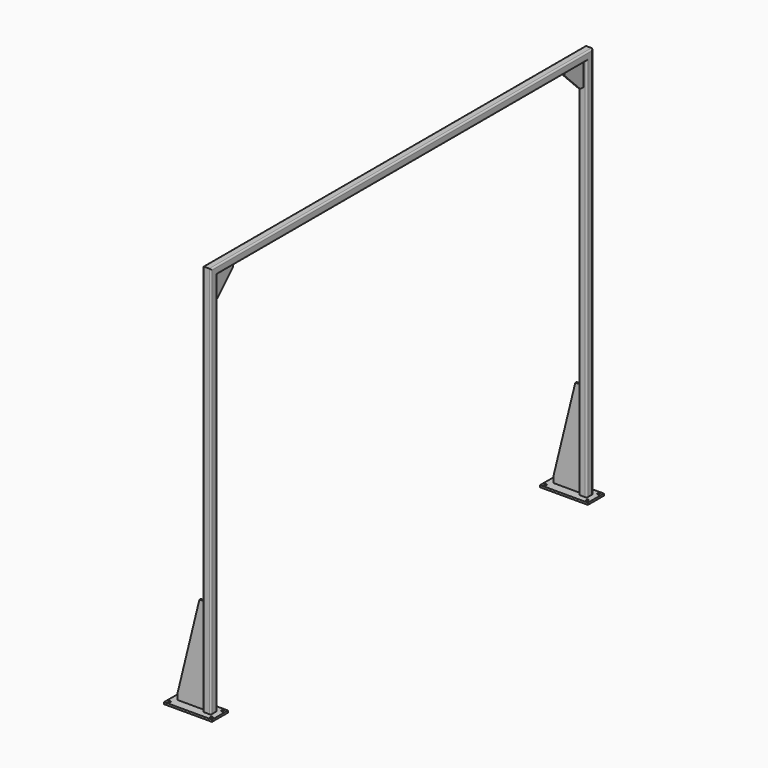
from build123d import *

# Parameters (mm, degrees)
F3_W      = 127
F3_H      = 127
F3_W_2    = 177.8
F4_DEPTH  = 12.7
F6_W      = 38.1
F6_H      = 38.1
F6_W_2    = 139.7
F6_H_2    = 571.5
F7_DEPTH  = 4.826
F9_D      = 14.2875
F13_DEPTH = 4.7625


# Not quite as in the source:
# - a length typed as a fraction of an inch, garbled in the dataset ("3 / 203.2 mm" for 3/8 in), is restored


with BuildPart() as f2:
    # F2: sweep along a path in F0
    with BuildLine(Plane.YZ) as f2_path:
        Line((-1524, 0), (-1524, 2501.9))
        Line((-1524, 2501.9), (1524, 2501.9))
        Line((1524, 2501.9), (1524, 0))
    # F1 (on Top) → F2 (sweep)
    with BuildSketch(Plane.XY):
        with BuildLine():
            Line((-15.748, -1524), (0, -1524))
            Line((0, -1524), (15.748, -1524))
            ThreePointArc((15.748, -1524), (22.572994652, -1521.172994652), (25.4, -1514.348))
            Line((25.4, -1514.348), (25.4, -1482.852))
            ThreePointArc((25.4, -1482.852), (22.572994652, -1476.027005348), (15.748, -1473.2))
            Line((15.748, -1473.2), (-15.748, -1473.2))
            ThreePointArc((-15.748, -1473.2), (-22.572994652, -1476.027005348), (-25.4, -1482.852))
            Line((-25.4, -1482.852), (-25.4, -1514.348))
            ThreePointArc((-25.4, -1514.348), (-22.572994652, -1521.172994652), (-15.748, -1524))
        make_face()
        with BuildLine():
            Line((0, -1519.2375), (-15.748, -1519.2375))
            ThreePointArc((-15.748, -1519.2375), (-19.2053986066, -1517.8053986066), (-20.6375, -1514.348))
            Line((-20.6375, -1514.348), (-20.6375, -1482.852))
            ThreePointArc((-20.6375, -1482.852), (-19.2053986066, -1479.3946013934), (-15.748, -1477.9625))
            Line((-15.748, -1477.9625), (15.748, -1477.9625))
            ThreePointArc((15.748, -1477.9625), (19.2053986066, -1479.3946013934), (20.6375, -1482.852))
            Line((20.6375, -1482.852), (20.6375, -1514.348))
            ThreePointArc((20.6375, -1514.348), (19.2053986066, -1517.8053986066), (15.748, -1519.2375))
            Line((15.748, -1519.2375), (0, -1519.2375))
        make_face(mode=Mode.SUBTRACT)
    sweep(path=f2_path.line, transition=Transition.RIGHT)

    # F3 (on face) → F4 (join)
    with BuildSketch(Plane(origin=(0, 0, 0), x_dir=(1, 0, 0), z_dir=(0, 0, -1))):
        with Locations((0, 1498.6)):
            Rectangle(F3_W, F3_H)
        with Locations((-152.4, 1498.6)):
            Rectangle(F3_W_2, F3_H)
    extrude(amount=F4_DEPTH)

    # F6 (on mid) → F7 (join, symmetric)
    with BuildSketch(Plane(origin=(0, -1498.6, 0), x_dir=(-1, 0, 0), z_dir=(0, 1, 0))):
        with Locations((44.45, 19.05)):
            Rectangle(F6_W, F6_H)
        with Locations((133.35, 19.05)):
            Rectangle(F6_W_2, F6_H)
        with Locations((44.45, 323.85)):
            Rectangle(F6_W, F6_H_2)
        Polygon((63.5, 609.6), (63.5, 38.1), (203.2, 38.1), align=None)
    extrude(amount=F7_DEPTH, both=True)

    # F9 (through all)
    with Locations(Plane(origin=(0, 0, -12.7), x_dir=(1, 0, 0), z_dir=(0, 0, -1))):
        with Locations((-222.25, 1454.15), (-222.25, 1543.05), (44.45, 1543.05), (44.45, 1454.15)):
            Hole(F9_D / 2)

    # F10: F2 across plane


with BuildPart() as f2_1:
    add(f2.part)
    add(f2.part.mirror(Plane.XZ))

    # F12 (on mid) → F13 (join, symmetric)
    with BuildSketch(Plane.YZ):
        Polygon((-1320.8, 2451.1), (-1473.2, 2451.1), (-1473.2, 2298.7), (-1447.8, 2298.7), (-1320.8, 2425.7), align=None)
    extrude(amount=F13_DEPTH, both=True)

    # F14: F2 across plane


with BuildPart() as f2_2:
    add(f2_1.part)
    add(f2_1.part.mirror(Plane.XZ))


solid = f2_2.part
